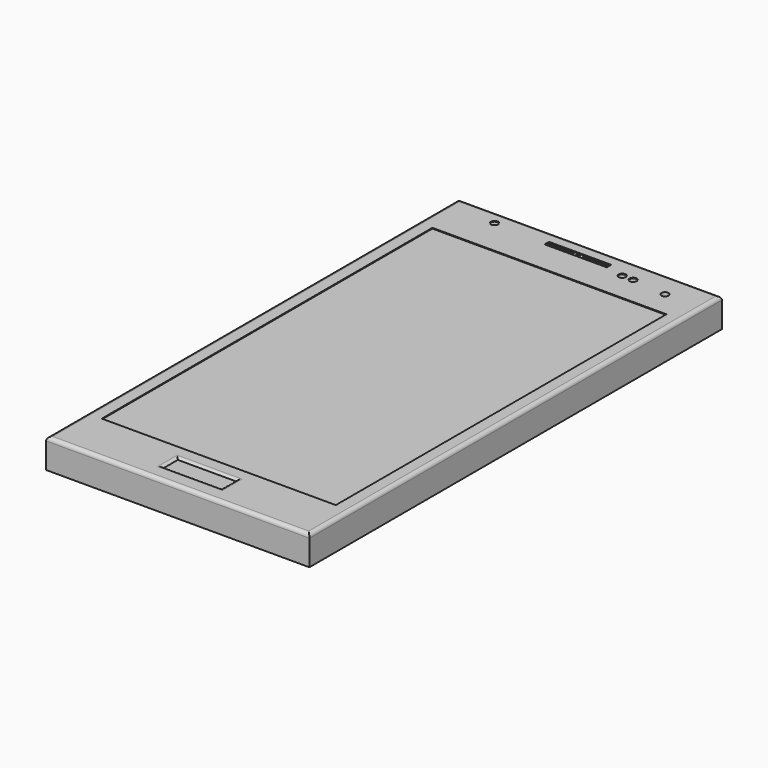
from build123d import *

# Parameters (mm, degrees)
F1_W         = 72
F1_H         = 141
F2_DEPTH     = 8
F0_R         = 1
F3_DEPTH     = 0.2
F0_W         = 64
F0_H         = 113
F0_W_2       = 17
F0_H_2       = 1.5
F0_R_2       = 0.5
F4_DEPTH     = 0.2
F5_DEPTH     = 0.5
F1_R         = 1
F6_DEPTH     = 2
F0_W_3       = 16
F0_H_3       = 5
F7_DEPTH     = 0.5
F8_T1_DEPTH  = 77
F8_T3_DEPTH  = 146
F8_T5_DEPTH  = 16
F8_T7_DEPTH  = 5
F8_T13_DEPTH = 7.1650635095
F8_T17_DEPTH = 18.1650635095
F8_T24_DEPTH = 18.1650635095
F8_T28_DEPTH = 7.1650635095
F8_T35_DEPTH = 7.1650635095
F8_T39_DEPTH = 18.1650635095
F8_T46_DEPTH = 7.1650635095
F8_T50_DEPTH = 18.1650635095


# Not quite as in the source:
# - a fillet or chamfer that OpenCascade refuses, or shapes differently, is made with other operations: its cross-section is extruded or revolved along the edge and cut away or added


with BuildPart() as f2:
    # F1 (on face) → F2 (new body)
    with BuildSketch(Plane.XY):
        with Locations((-0.0423140228, 0.0165017247)):
            Rectangle(F1_W, F1_H)
    extrude(amount=-F2_DEPTH)

    # F0 (on Top) → F3 (cut)
    with BuildSketch(Plane.XY):
        with Locations((-23, 66.5)):
            Circle(F0_R)
        with Locations((13.5, 64.5)):
            Circle(F0_R)
        with Locations((16.5, 64.5)):
            Circle(F0_R)
    extrude(amount=-F3_DEPTH, mode=Mode.SUBTRACT)

    # F0 (on Top) → F4 (cut)
    with BuildSketch(Plane.XY):
        Rectangle(F0_W, F0_H)
        with Locations((0, 66.2368237972)):
            Rectangle(F0_W_2, F0_H_2)
        with Locations((-7.8863224118, 66.2359703599)):
            Circle(F0_R_2, mode=Mode.SUBTRACT)
        with Locations((-6.75, 66.25)):
            Circle(F0_R_2, mode=Mode.SUBTRACT)
        with Locations((-5.5, 66.25)):
            Circle(F0_R_2, mode=Mode.SUBTRACT)
        with Locations((-4.25, 66.2368237972)):
            Circle(F0_R_2, mode=Mode.SUBTRACT)
        with Locations((-3, 66.25)):
            Circle(F0_R_2, mode=Mode.SUBTRACT)
        with Locations((-1.75, 66.25)):
            Circle(F0_R_2, mode=Mode.SUBTRACT)
        with BuildLine():
            ThreePointArc((0, 65.7368237972), (-0.3535533906, 66.5903771878), (0.5, 66.2368237972))
            ThreePointArc((0.5, 66.2368237972), (0.3535533906, 65.8832704066), (0, 65.7368237972))
        make_face(mode=Mode.SUBTRACT)
        with Locations((1.75, 66.25)):
            Circle(F0_R_2, mode=Mode.SUBTRACT)
        with Locations((3, 66.25)):
            Circle(F0_R_2, mode=Mode.SUBTRACT)
        with Locations((4.25, 66.2368237972)):
            Circle(F0_R_2, mode=Mode.SUBTRACT)
        with Locations((5.5, 66.25)):
            Circle(F0_R_2, mode=Mode.SUBTRACT)
        with Locations((6.75, 66.25)):
            Circle(F0_R_2, mode=Mode.SUBTRACT)
        with Locations((7.8863224118, 66.2359703599)):
            Circle(F0_R_2, mode=Mode.SUBTRACT)
    extrude(amount=-F4_DEPTH, mode=Mode.SUBTRACT)

    # F0 (on Top) → F5 (cut)
    with BuildSketch(Plane.XY):
        with Locations((-7.8863224118, 66.2359703599)):
            Circle(F0_R_2)
        with Locations((-6.75, 66.25)):
            Circle(F0_R_2)
        with Locations((1.75, 66.25)):
            Circle(F0_R_2)
        with Locations((3, 66.25)):
            Circle(F0_R_2)
        with BuildLine():
            ThreePointArc((0, 65.7368237972), (0.3535533906, 65.8832704066), (0.5, 66.2368237972))
            ThreePointArc((0.5, 66.2368237972), (-0.3535533906, 66.5903771878), (0, 65.7368237972))
        make_face()
        with Locations((-4.25, 66.2368237972)):
            Circle(F0_R_2)
        with Locations((-3, 66.25)):
            Circle(F0_R_2)
        with Locations((-1.75, 66.25)):
            Circle(F0_R_2)
        with Locations((4.25, 66.2368237972)):
            Circle(F0_R_2)
        with Locations((5.5, 66.25)):
            Circle(F0_R_2)
        with Locations((6.75, 66.25)):
            Circle(F0_R_2)
        with Locations((7.8863224118, 66.2359703599)):
            Circle(F0_R_2)
        with Locations((-5.5, 66.25)):
            Circle(F0_R_2)
    extrude(amount=-F5_DEPTH, mode=Mode.SUBTRACT)

    # F1 (on face) → F6 (cut)
    with BuildSketch(Plane.XY):
        with Locations((26.0005407035, 63.5057538748)):
            Circle(F1_R)
    extrude(amount=-F6_DEPTH, mode=Mode.SUBTRACT)

    # F0 (on Top) → F7 (cut)
    with BuildSketch(Plane.XY):
        with Locations((0, -63)):
            Rectangle(F0_W_3, F0_H_3)
    extrude(amount=-F7_DEPTH, mode=Mode.SUBTRACT)

    # F8: fillet of radius 1 on 8 edges, made by hand

    # F8_s2 → F8_t1 (cut)
    with BuildSketch(Plane.YZ.offset(-38.5423140228)):
        with BuildLine():
            ThreePointArc((70.5165017247, -1), (70.2236085059, -0.2928932188), (69.5165017247, 0))
            Line((69.5165017247, 0), (70.5165017247, 0))
            Line((70.5165017247, 0), (70.5165017247, -1))
        make_face()
        with BuildLine():
            ThreePointArc((-70.4834982753, -1), (-70.1906050565, -0.2928932188), (-69.4834982753, 0))
            Line((-69.4834982753, 0), (-70.4834982753, 0))
            Line((-70.4834982753, 0), (-70.4834982753, -1))
        make_face()
    extrude(amount=F8_T1_DEPTH, mode=Mode.SUBTRACT)

    # F8_s4 → F8_t3 (cut)
    with BuildSketch(Plane.XZ.offset(-73.0165017247)):
        with BuildLine():
            ThreePointArc((-35.0423140228, 0), (-35.749420804, -0.2928932188), (-36.0423140228, -1))
            Line((-36.0423140228, -1), (-36.0423140228, 0))
            Line((-36.0423140228, 0), (-35.0423140228, 0))
        make_face()
        with BuildLine():
            ThreePointArc((35.9576859772, -1), (35.6647927584, -0.2928932188), (34.9576859772, 0))
            Line((34.9576859772, 0), (35.9576859772, 0))
            Line((35.9576859772, 0), (35.9576859772, -1))
        make_face()
    extrude(amount=F8_T3_DEPTH, mode=Mode.SUBTRACT)

    # F8_s6 → F8_t5 (cut)
    with BuildSketch(Plane.YZ.offset(-8)):
        with BuildLine():
            ThreePointArc((-59.6339745962, 0), (-60.1339745962, -0.1339745962), (-60.5, -0.5))
            Line((-60.5, -0.5), (-60.5, 0))
            Line((-60.5, 0), (-59.6339745962, 0))
        make_face()
        with BuildLine():
            ThreePointArc((-66.3660254038, 0), (-65.8660254038, -0.1339745962), (-65.5, -0.5))
            Line((-65.5, -0.5), (-65.5, 0))
            Line((-65.5, 0), (-66.3660254038, 0))
        make_face()
    extrude(amount=F8_T5_DEPTH, mode=Mode.SUBTRACT)

    # F8_s8 → F8_t7 (cut)
    with BuildSketch(Plane.XZ.offset(60.5)):
        with BuildLine():
            ThreePointArc((-8.8660254038, 0), (-8.3660254038, -0.1339745962), (-8, -0.5))
            Line((-8, -0.5), (-8, 0))
            Line((-8, 0), (-8.8660254038, 0))
        make_face()
        with BuildLine():
            ThreePointArc((8.8660254038, 0), (8.3660254038, -0.1339745962), (8, -0.5))
            Line((8, -0.5), (8, 0))
            Line((8, 0), (8.8660254038, 0))
        make_face()
    extrude(amount=F8_T7_DEPTH, mode=Mode.SUBTRACT)


with BuildPart() as f8_tool11:
    # F8_s12 → F8_t13 (new body)
    with BuildSketch(Plane.XZ.offset(65.5)):
        with BuildLine():
            ThreePointArc((8.8660254038, 0), (8.3660254038, -0.1339745962), (8, -0.5))
            Line((8, -0.5), (8, 0))
            Line((8, 0), (8.8660254038, 0))
        make_face()
    extrude(amount=-F8_T13_DEPTH)

    split(bisect_by=Plane.XZ.offset(60.5), keep=Keep.BOTTOM)


with BuildPart() as f8_tool15:
    # F8_s16 → F8_t17 (new body)
    with BuildSketch(Plane.YZ.offset(10.1650635095)):
        with BuildLine():
            ThreePointArc((-59.6339745962, 0), (-60.1339745962, -0.1339745962), (-60.5, -0.5))
            Line((-60.5, -0.5), (-60.5, 0))
            Line((-60.5, 0), (-59.6339745962, 0))
        make_face()
    extrude(amount=-F8_T17_DEPTH)

    split(bisect_by=Plane.YZ.offset(8), keep=Keep.TOP)


with BuildPart() as f8_tool11_1:
    add(f8_tool11.part)

    # F8_t19: intersect F8_tool15
    add(f8_tool15.part, mode=Mode.INTERSECT)


with BuildPart() as f2_1:
    add(f2.part)

    # F8_t9: cut F8_tool11
    add(f8_tool11_1.part, mode=Mode.SUBTRACT)


with BuildPart() as f8_tool22:
    # F8_s23 → F8_t24 (new body)
    with BuildSketch(Plane.YZ.offset(8)):
        with BuildLine():
            ThreePointArc((-59.6339745962, 0), (-60.1339745962, -0.1339745962), (-60.5, -0.5))
            Line((-60.5, -0.5), (-60.5, 0))
            Line((-60.5, 0), (-59.6339745962, 0))
        make_face()
    extrude(amount=-F8_T24_DEPTH)

    split(bisect_by=Plane.YZ.offset(-8), keep=Keep.BOTTOM)


with BuildPart() as f8_tool26:
    # F8_s27 → F8_t28 (new body)
    with BuildSketch(Plane.XZ.offset(58.3349364905)):
        with BuildLine():
            ThreePointArc((-8.8660254038, 0), (-8.3660254038, -0.1339745962), (-8, -0.5))
            Line((-8, -0.5), (-8, 0))
            Line((-8, 0), (-8.8660254038, 0))
        make_face()
    extrude(amount=F8_T28_DEPTH)

    split(bisect_by=Plane.XZ.offset(60.5), keep=Keep.BOTTOM)


with BuildPart() as f8_tool22_1:
    add(f8_tool22.part)

    # F8_t30: intersect F8_tool26
    add(f8_tool26.part, mode=Mode.INTERSECT)


with BuildPart() as f2_2:
    add(f2_1.part)

    # F8_t20: cut F8_tool22
    add(f8_tool22_1.part, mode=Mode.SUBTRACT)


with BuildPart() as f8_tool33:
    # F8_s34 → F8_t35 (new body)
    with BuildSketch(Plane.XZ.offset(60.5)):
        with BuildLine():
            ThreePointArc((-8.8660254038, 0), (-8.3660254038, -0.1339745962), (-8, -0.5))
            Line((-8, -0.5), (-8, 0))
            Line((-8, 0), (-8.8660254038, 0))
        make_face()
    extrude(amount=F8_T35_DEPTH)

    split(bisect_by=Plane.XZ.offset(65.5), keep=Keep.TOP)


with BuildPart() as f8_tool37:
    # F8_s38 → F8_t39 (new body)
    with BuildSketch(Plane.YZ.offset(-10.1650635095)):
        with BuildLine():
            ThreePointArc((-66.3660254038, 0), (-65.8660254038, -0.1339745962), (-65.5, -0.5))
            Line((-65.5, -0.5), (-65.5, 0))
            Line((-65.5, 0), (-66.3660254038, 0))
        make_face()
    extrude(amount=F8_T39_DEPTH)

    split(bisect_by=Plane.YZ.offset(-8), keep=Keep.BOTTOM)


with BuildPart() as f8_tool33_1:
    add(f8_tool33.part)

    # F8_t41: intersect F8_tool37
    add(f8_tool37.part, mode=Mode.INTERSECT)


with BuildPart() as f2_3:
    add(f2_2.part)

    # F8_t31: cut F8_tool33
    add(f8_tool33_1.part, mode=Mode.SUBTRACT)


with BuildPart() as f8_tool44:
    # F8_s45 → F8_t46 (new body)
    with BuildSketch(Plane.XZ.offset(67.6650635095)):
        with BuildLine():
            ThreePointArc((8.8660254038, 0), (8.3660254038, -0.1339745962), (8, -0.5))
            Line((8, -0.5), (8, 0))
            Line((8, 0), (8.8660254038, 0))
        make_face()
    extrude(amount=-F8_T46_DEPTH)

    split(bisect_by=Plane.XZ.offset(65.5), keep=Keep.TOP)


with BuildPart() as f8_tool48:
    # F8_s49 → F8_t50 (new body)
    with BuildSketch(Plane.YZ.offset(-8)):
        with BuildLine():
            ThreePointArc((-66.3660254038, 0), (-65.8660254038, -0.1339745962), (-65.5, -0.5))
            Line((-65.5, -0.5), (-65.5, 0))
            Line((-65.5, 0), (-66.3660254038, 0))
        make_face()
    extrude(amount=F8_T50_DEPTH)

    split(bisect_by=Plane.YZ.offset(8), keep=Keep.TOP)


with BuildPart() as f8_tool44_1:
    add(f8_tool44.part)

    # F8_t52: intersect F8_tool48
    add(f8_tool48.part, mode=Mode.INTERSECT)


with BuildPart() as f2_4:
    add(f2_3.part)

    # F8_t42: cut F8_tool44
    add(f8_tool44_1.part, mode=Mode.SUBTRACT)


solid = f2_4.part
